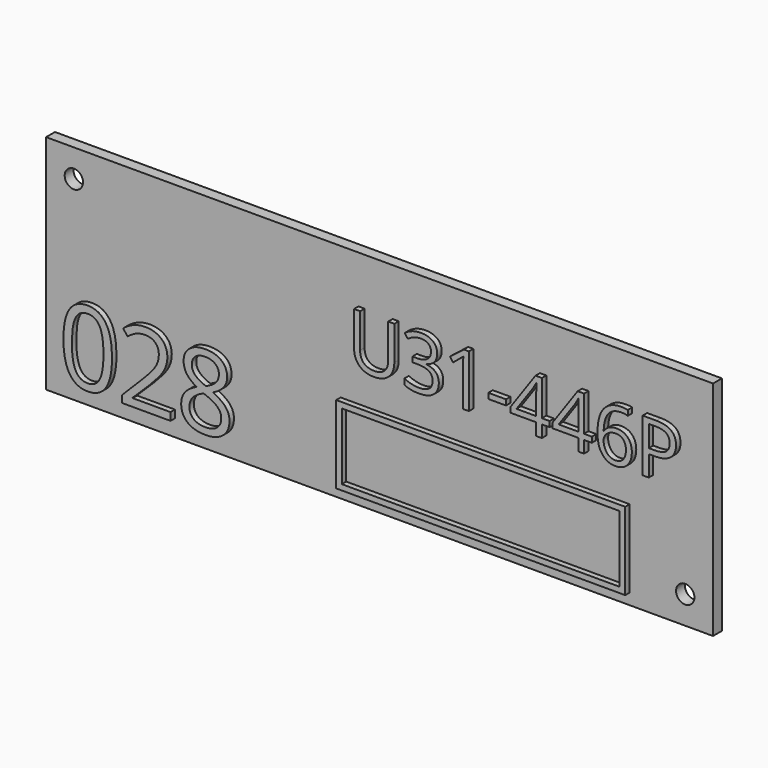
from build123d import *

# Parameters (mm, degrees)
F0_W         = 120
F0_H         = 40
F1_DEPTH     = 2
F3_D         = 3.3
F4_TEXT_SIZE = 13.2628743135
F5_DEPTH     = 1
F6_TEXT_SIZE = 18.5155049272
F7_DEPTH     = 1
F8_W         = 52
F8_H         = 14
F8_W_2       = 49.99999962
F8_H_2       = 11.99999962
F9_DEPTH     = 1


# Not quite as in the source:
# - Text() gives the source's letters only with a copy of the font that has no kerning and outlines rounded to 1/6400 em; it was checked with that copy


with BuildPart() as f1:
    # F0 (on Front) → F1 (new body)
    with BuildSketch(Plane.XZ):
        Rectangle(F0_W, F0_H)
    extrude(amount=F1_DEPTH)

    # F3 (through all)
    with Locations(Plane.XZ.offset(2)):
        with Locations((-55, 15), (55, -15)):
            Hole(F3_D / 2)

    # F4 (on face) → F5 (join)
    with BuildSketch(Plane.XZ.offset(2)):
        with Locations((-5, 2)):
            Text('U31-446P', F4_TEXT_SIZE, font='Open Sans', text_align=(TextAlign.LEFT, TextAlign.BOTTOM))
    extrude(amount=F5_DEPTH)

    # F6 (on face) → F7 (join)
    with BuildSketch(Plane.XZ.offset(2)):
        with Locations((-57, -17)):
            Text('028', F6_TEXT_SIZE, font='Open Sans', text_align=(TextAlign.LEFT, TextAlign.BOTTOM))
    extrude(amount=F7_DEPTH)

    # F8 (on face) → F9 (join)
    with BuildSketch(Plane.XZ.offset(2)):
        with Locations((19, -11)):
            Rectangle(F8_W, F8_H)
        with Locations((19, -11)):
            Rectangle(F8_W_2, F8_H_2, mode=Mode.SUBTRACT)
    extrude(amount=F9_DEPTH)


solid = f1.part
